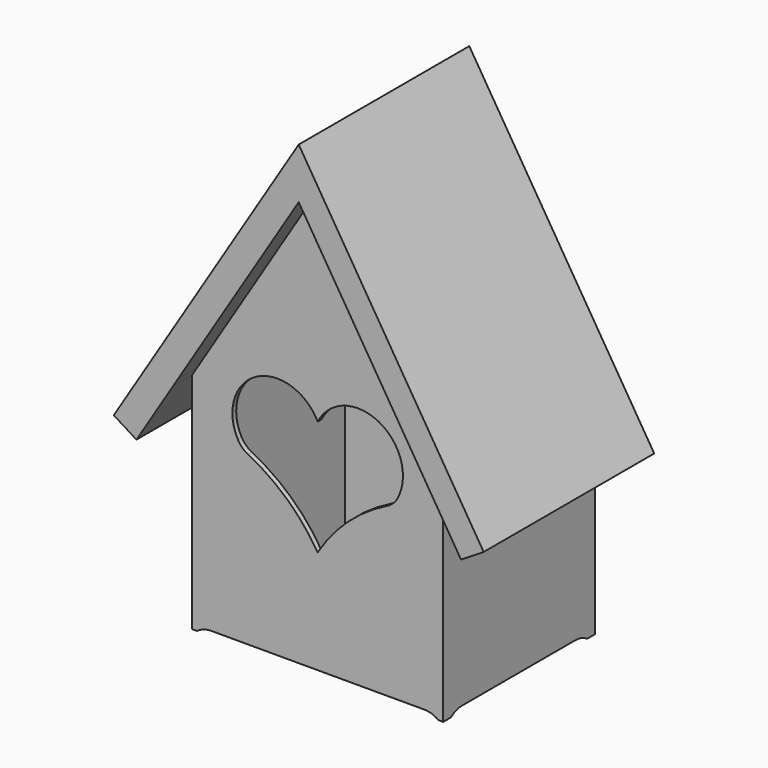
from build123d import *

# Parameters (mm, degrees)
F0_W         = 50.964426635
F0_H         = 1
F1_DEPTH     = 40
F2_DEPTH     = 45
F3_DEPTH     = 5
F4_START     = 1
F4_DEPTH     = 44.001
F6_START     = 1
F6_DEPTH     = 38
F7_START     = 1
F7_DEPTH     = 44.001
F9_DEPTH     = 25
F11_DEPTH    = 25
F12_T1_DEPTH = 1
F12_T3_DEPTH = 1


# Not quite as in the source:
# - a fillet or chamfer that OpenCascade refuses, or shapes differently, is made with other operations: its cross-section is extruded or revolved along the edge and cut away or added


with BuildPart() as f1:
    # F0 (on Front) → F1 (new body)
    with BuildSketch(Plane.XZ):
        Polygon((25.4822133175, 48.8744375096), (0, 90), (-25.4822133175, 48.8744375096), (-25.4822133175, 1), (25.4822133175, 1), align=None)
        with BuildLine():
            ThreePointArc((-16.8351454988, 38.3754507383), (-12.9010914993, 51.3524985976), (0, 47.1760898363))
            ThreePointArc((0, 47.1760898363), (12.8897582031, 51.3584134172), (16.847382477, 38.3979000332))
            ThreePointArc((16.847382477, 38.3979000332), (15.916282128, 37.1777103045), (14.6589247027, 36.2974471967))
            ThreePointArc((14.6589247027, 36.2974471967), (6.3677193864, 30.6369091459), (0, 22.8755995631))
            ThreePointArc((0, 22.8755995631), (-6.3946665322, 30.6177021843), (-14.6752906719, 36.297770574))
            ThreePointArc((-14.6752906719, 36.297770574), (-15.914547628, 37.1709794451), (-16.8351454988, 38.3754507383))
        make_face(mode=Mode.SUBTRACT)
        with BuildLine():
            Line((-2.5, 73.7544666829), (-2.5, 77.2864818573))
            ThreePointArc((-2.5, 77.2864818573), (0, 79.7864818573), (2.5, 77.2864818573))
            Line((2.5, 77.2864818573), (2.5, 73.7544666829))
            ThreePointArc((2.5, 73.7544666829), (0, 67.8049769402), (-2.5, 73.7544666829))
        make_face(mode=Mode.SUBTRACT)
        with BuildLine():
            ThreePointArc((16.847382477, 38.3979000332), (12.8897582031, 51.3584134172), (0, 47.1760898363))
            ThreePointArc((0, 47.1760898363), (-12.9010914993, 51.3524985976), (-16.8351454988, 38.3754507383))
            ThreePointArc((-16.8351454988, 38.3754507383), (-15.914547628, 37.1709794451), (-14.6752906719, 36.297770574))
            ThreePointArc((-14.6752906719, 36.297770574), (-6.3946665322, 30.6177021843), (0, 22.8755995631))
            ThreePointArc((0, 22.8755995631), (6.3677193864, 30.6369091459), (14.6589247027, 36.2974471967))
            ThreePointArc((14.6589247027, 36.2974471967), (15.916282128, 37.1777103045), (16.847382477, 38.3979000332))
        make_face()
        with BuildLine():
            ThreePointArc((2.5, 77.2864818573), (0, 79.7864818573), (-2.5, 77.2864818573))
            Line((-2.5, 77.2864818573), (-2.5, 73.7544666829))
            ThreePointArc((-2.5, 73.7544666829), (0, 67.8049769402), (2.5, 73.7544666829))
            Line((2.5, 73.7544666829), (2.5, 77.2864818573))
        make_face()
        with Locations((0, 0.5)):
            Rectangle(F0_W, F0_H)
        Polygon((-25.4822133175, 1), (-25.4822133175, 48.8744375096), (-26.4822133175, 47.2605446354), (-26.4822133175, 0), (-25.4822133175, 0), align=None)
        Polygon((26.4822133175, 47.2605446354), (25.4822133175, 48.8744375096), (25.4822133175, 1), (25.4822133175, 0), (26.4822133175, 0), align=None)
    extrude(amount=F1_DEPTH)

    # F0 (on Front) → F2 (join)
    with BuildSketch(Plane.XZ):
        Polygon((-26.4822133175, 47.2605446354), (-25.4822133175, 48.8744375096), (-25.4822133175, 50.7730291479), (-34.5699527606, 36.1063912187), (-37.6622251316, 38.0224244453), (-25.4822133175, 57.679658719), (0, 98.8052212095), (25.4822133175, 57.679658719), (37.6622251316, 38.0224244453), (34.5699527606, 36.1063912187), (25.4822133175, 50.7730291479), (25.4822133175, 48.8744375096), (26.4822133175, 47.2605446354), (34.2466115735, 34.7296376181), (39.0389787322, 37.6990832582), (0, 100.7038128478), (-39.0389787322, 37.6990832582), (-34.2466115735, 34.7296376181), align=None)
        Polygon((-25.4822133175, 48.8744375096), (0, 90), (25.4822133175, 48.8744375096), (25.4822133175, 50.7730291479), (25.4822133175, 57.679658719), (0, 98.8052212095), (-25.4822133175, 57.679658719), (-25.4822133175, 50.7730291479), align=None)
        Polygon((-34.5699527606, 36.1063912187), (-25.4822133175, 50.7730291479), (-25.4822133175, 57.679658719), (-37.6622251316, 38.0224244453), align=None)
        Polygon((25.4822133175, 57.679658719), (25.4822133175, 50.7730291479), (34.5699527606, 36.1063912187), (37.6622251316, 38.0224244453), align=None)
    extrude(amount=F2_DEPTH)

    # F0 (on Front) → F3 (cut)
    with BuildSketch(Plane.XZ):
        with BuildLine():
            ThreePointArc((2.5, 77.2864818573), (0, 79.7864818573), (-2.5, 77.2864818573))
            Line((-2.5, 77.2864818573), (-2.5, 73.7544666829))
            ThreePointArc((-2.5, 73.7544666829), (0, 67.8049769402), (2.5, 73.7544666829))
            Line((2.5, 73.7544666829), (2.5, 77.2864818573))
        make_face()
        with Locations((0, 0.5)):
            Rectangle(F0_W, F0_H)
    extrude(amount=F3_DEPTH, mode=Mode.SUBTRACT)

    # F0 (on Front) → F4 (cut)
    with BuildSketch(Plane.XZ.offset(F4_START)):
        with BuildLine():
            ThreePointArc((16.847382477, 38.3979000332), (12.8897582031, 51.3584134172), (0, 47.1760898363))
            ThreePointArc((0, 47.1760898363), (-12.9010914993, 51.3524985976), (-16.8351454988, 38.3754507383))
            ThreePointArc((-16.8351454988, 38.3754507383), (-15.914547628, 37.1709794451), (-14.6752906719, 36.297770574))
            ThreePointArc((-14.6752906719, 36.297770574), (-6.3946665322, 30.6177021843), (0, 22.8755995631))
            ThreePointArc((0, 22.8755995631), (6.3677193864, 30.6369091459), (14.6589247027, 36.2974471967))
            ThreePointArc((14.6589247027, 36.2974471967), (15.916282128, 37.1777103045), (16.847382477, 38.3979000332))
        make_face()
    extrude(amount=F4_DEPTH, mode=Mode.SUBTRACT)

    # F0 (on Front) → F6 (cut)
    with BuildSketch(Plane.XZ.offset(F6_START)):
        Polygon((25.4822133175, 48.8744375096), (0, 90), (-25.4822133175, 48.8744375096), (-25.4822133175, 1), (25.4822133175, 1), align=None)
        with BuildLine():
            ThreePointArc((-16.8351454988, 38.3754507383), (-12.9010914993, 51.3524985976), (0, 47.1760898363))
            ThreePointArc((0, 47.1760898363), (12.8897582031, 51.3584134172), (16.847382477, 38.3979000332))
            ThreePointArc((16.847382477, 38.3979000332), (15.916282128, 37.1777103045), (14.6589247027, 36.2974471967))
            ThreePointArc((14.6589247027, 36.2974471967), (6.3677193864, 30.6369091459), (0, 22.8755995631))
            ThreePointArc((0, 22.8755995631), (-6.3946665322, 30.6177021843), (-14.6752906719, 36.297770574))
            ThreePointArc((-14.6752906719, 36.297770574), (-15.914547628, 37.1709794451), (-16.8351454988, 38.3754507383))
        make_face(mode=Mode.SUBTRACT)
        with BuildLine():
            Line((-2.5, 73.7544666829), (-2.5, 77.2864818573))
            ThreePointArc((-2.5, 77.2864818573), (0, 79.7864818573), (2.5, 77.2864818573))
            Line((2.5, 77.2864818573), (2.5, 73.7544666829))
            ThreePointArc((2.5, 73.7544666829), (0, 67.8049769402), (-2.5, 73.7544666829))
        make_face(mode=Mode.SUBTRACT)
        Polygon((-25.4822133175, 48.8744375096), (0, 90), (25.4822133175, 48.8744375096), (25.4822133175, 50.7730291479), (25.4822133175, 57.679658719), (0, 98.8052212095), (-25.4822133175, 57.679658719), (-25.4822133175, 50.7730291479), align=None)
        with BuildLine():
            ThreePointArc((2.5, 77.2864818573), (0, 79.7864818573), (-2.5, 77.2864818573))
            Line((-2.5, 77.2864818573), (-2.5, 73.7544666829))
            ThreePointArc((-2.5, 73.7544666829), (0, 67.8049769402), (2.5, 73.7544666829))
            Line((2.5, 73.7544666829), (2.5, 77.2864818573))
        make_face()
        Polygon((-34.5699527606, 36.1063912187), (-25.4822133175, 50.7730291479), (-25.4822133175, 57.679658719), (-37.6622251316, 38.0224244453), align=None)
        Polygon((25.4822133175, 57.679658719), (25.4822133175, 50.7730291479), (34.5699527606, 36.1063912187), (37.6622251316, 38.0224244453), align=None)
        with Locations((0, 0.5)):
            Rectangle(F0_W, F0_H)
    extrude(amount=F6_DEPTH, mode=Mode.SUBTRACT)

    # F0 (on Front) → F7 (cut)
    with BuildSketch(Plane.XZ.offset(F7_START)):
        with Locations((0, 0.5)):
            Rectangle(F0_W, F0_H)
    extrude(amount=F7_DEPTH, mode=Mode.SUBTRACT)

    # F8 (on face) → F9 (cut)
    with BuildSketch(Plane(origin=(-26.4822133175, 0, 0), x_dir=(0, -1, 0), z_dir=(-1, 0, 0))):
        with BuildLine():
            Line((34.9282032303, 1), (5.0717967697, 1))
            ThreePointArc((5.0717967697, 1), (3.7777015442, 0.8296291314), (2.5717967697, 0.3301270189))
            Line((2.5717967697, 0.3301270189), (2, 0))
            Line((2, 0), (38, 0))
            Line((38, 0), (37.4282032303, 0.3301270189))
            ThreePointArc((37.4282032303, 0.3301270189), (36.2222984558, 0.8296291314), (34.9282032303, 1))
        make_face()
    extrude(amount=-F9_DEPTH, mode=Mode.SUBTRACT)

    # F10 (on face) → F11 (cut)
    with BuildSketch(Plane.YZ.offset(26.4822133175)):
        with BuildLine():
            Line((-37.4282032303, 0.3301270189), (-38, 0))
            Line((-38, 0), (-2, 0))
            Line((-2, 0), (-2.5717967697, 0.3301270189))
            ThreePointArc((-2.5717967697, 0.3301270189), (-3.7777015442, 0.8296291314), (-5.0717967697, 1))
            Line((-5.0717967697, 1), (-34.9282032303, 1))
            ThreePointArc((-34.9282032303, 1), (-36.2222984558, 0.8296291314), (-37.4282032303, 0.3301270189))
        make_face()
    extrude(amount=-F11_DEPTH, mode=Mode.SUBTRACT)

    # F12: fillet of radius 5 on 4 edges, made by hand

    # F12_s2 → F12_t1 (join)
    with BuildSketch(Plane.XZ):
        with BuildLine():
            ThreePointArc((25.4822133175, 0), (24.0633521476, 0.7434164903), (22.4822133175, 1))
            Line((22.4822133175, 1), (25.4822133175, 1))
            Line((25.4822133175, 1), (25.4822133175, 0))
        make_face()
        with BuildLine():
            ThreePointArc((-22.4822133175, 1), (-24.0633521476, 0.7434164903), (-25.4822133175, 0))
            Line((-25.4822133175, 0), (-25.4822133175, 1))
            Line((-25.4822133175, 1), (-22.4822133175, 1))
        make_face()
    extrude(amount=F12_T1_DEPTH)

    # F12_s4 → F12_t3 (join)
    with BuildSketch(Plane.XZ.offset(39)):
        with BuildLine():
            ThreePointArc((25.4822133175, 0), (24.0633521476, 0.7434164903), (22.4822133175, 1))
            Line((22.4822133175, 1), (25.4822133175, 1))
            Line((25.4822133175, 1), (25.4822133175, 0))
        make_face()
        with BuildLine():
            ThreePointArc((-25.4822133175, 0), (-24.0633521476, 0.7434164903), (-22.4822133175, 1))
            Line((-22.4822133175, 1), (-25.4822133175, 1))
            Line((-25.4822133175, 1), (-25.4822133175, 0))
        make_face()
    extrude(amount=F12_T3_DEPTH)


solid = f1.part
